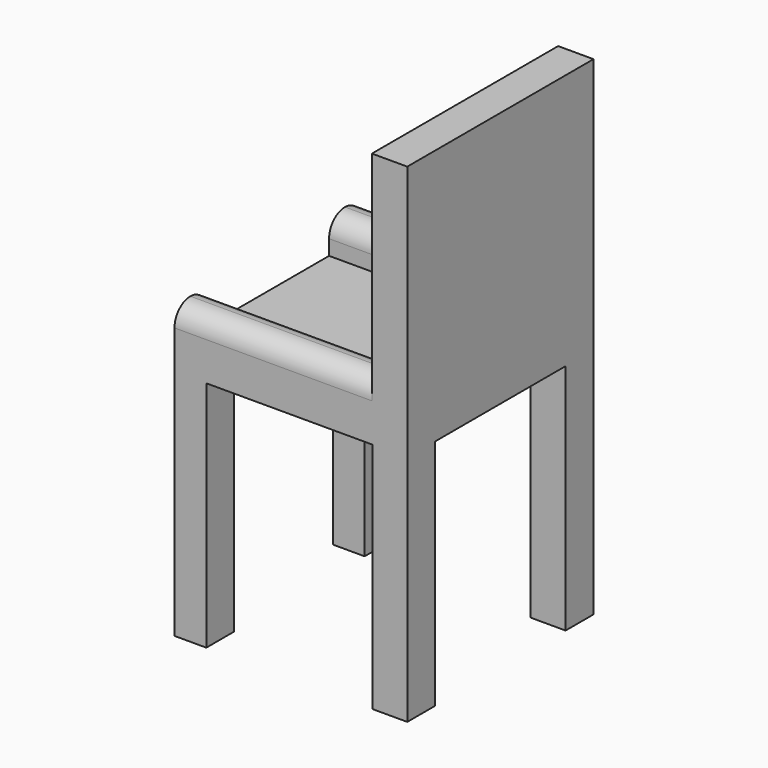
from build123d import *

# Parameters (mm, degrees)
F0_W      = 25.4
F0_H      = 25.4
F1_DEPTH  = 2.54
F2_W      = 3.4710424952
F2_H      = 3.81
F2_W_2    = 3.81
F3_DEPTH  = 25.4
F4_W      = 3.8600380808
F4_H      = 25.4
F5_DEPTH  = 25.4
F6_W      = 21.5399619192
F6_H      = 4.318
F7_DEPTH  = 3.81
F8_R      = 2.15899
F9_W      = 21.5399619192
F9_H      = 4.318
F10_DEPTH = 3.81
F11_R     = 2.159
F12_R     = 2.15899


# Not quite as in the source:
# - a fillet or chamfer is up to 0.001 mm smaller than in the source, because OpenCascade refuses the exact size


with BuildPart() as f1:
    # F0 (on Top) → F1 (new body)
    with BuildSketch(Plane.XY):
        with Locations((12.7, 12.7)):
            Rectangle(F0_W, F0_H)
    extrude(amount=F1_DEPTH)

    # F2 (on face) → F3 (join)
    with BuildSketch(Plane(origin=(0, 0, 0), x_dir=(1, 0, 0), z_dir=(0, 0, -1))):
        with Locations((1.7355212476, -1.905)):
            Rectangle(F2_W, F2_H)
        with Locations((23.495, -1.905)):
            Rectangle(F2_W_2, F2_H)
        with Locations((1.7355212476, -23.495)):
            Rectangle(F2_W, F2_H)
        with Locations((23.495, -23.495)):
            Rectangle(F2_W_2, F2_H)
    extrude(amount=F3_DEPTH)

    # F4 (on face) → F5 (join)
    with BuildSketch(Plane.XY.offset(2.54)):
        with Locations((23.4699809596, 12.7)):
            Rectangle(F4_W, F4_H)
    extrude(amount=F5_DEPTH)

    # F6 (on face) → F7 (join)
    with BuildSketch(Plane.XY.offset(2.54)):
        with Locations((10.7699809596, 23.241)):
            Rectangle(F6_W, F6_H)
    extrude(amount=F7_DEPTH)

    # F8 (radius 2.159 in the source; OpenCascade refuses exactly that, so slightly less here)
    f8_edges = [f1.edges().sort_by_distance(p)[0] for p in [
        (10.769981, 25.4, 6.35),
        (10.769981, 21.082, 6.35),
    ]]
    fillet(f8_edges, radius=F8_R)

    # F9 (on face) → F10 (join)
    with BuildSketch(Plane.XY.offset(2.54)):
        with Locations((10.7699809596, 2.159)):
            Rectangle(F9_W, F9_H)
    extrude(amount=F10_DEPTH)

    # F11
    f11_edges = [f1.edges().sort_by_distance(p)[0] for p in [
        (10.769981, 0, 6.35),
    ]]
    fillet(f11_edges, radius=F11_R)

    # F12 (radius 2.159 in the source; OpenCascade refuses exactly that, so slightly less here)
    f12_edges = [f1.edges().sort_by_distance(p)[0] for p in [
        (10.769981, 4.318, 6.35),
    ]]
    fillet(f12_edges, radius=F12_R)


solid = f1.part
